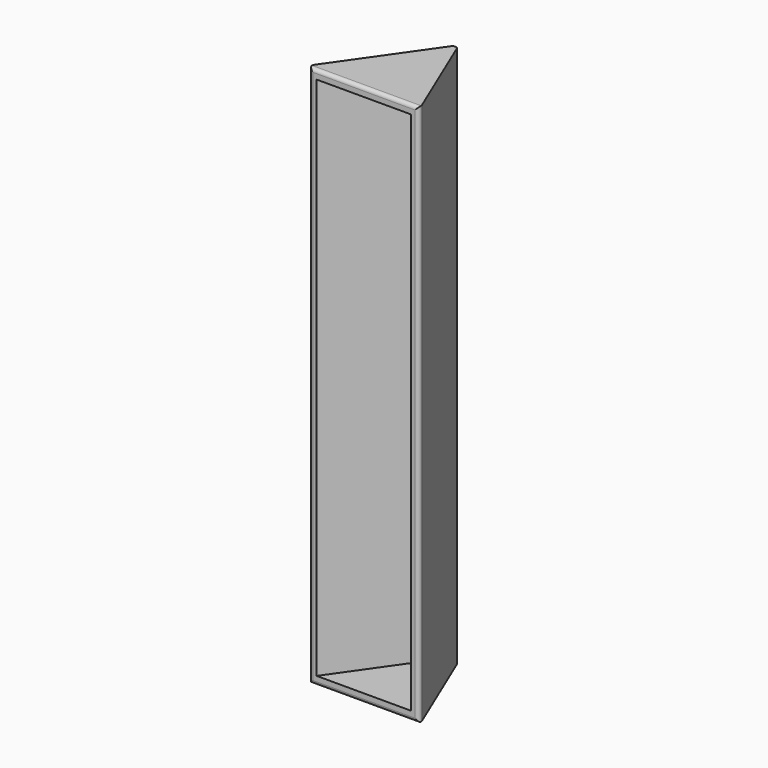
from build123d import *

# Parameters (mm, degrees)
F1_DEPTH      = 78.5
F2_T          = -2.5
F3_R          = 1
F4_TEXT_SIZE  = 12.5527115818
F5_DEPTH      = 1
F6_TEXT_SIZE  = 6.9016590714
F7_DEPTH      = 2
F8_TEXT_SIZE  = 8.8861462512
F9_DEPTH      = 1
F10_TEXT_SIZE = 8.2279131955
F11_DEPTH     = 0.5


# Not quite as in the source:
# - Text() gives the source's letters only with a copy of the font that has no kerning and outlines rounded to 1/6400 em; it was checked with that copy


with BuildPart() as f1:
    # F0 (on Top) → F1 (new body, symmetric)
    with BuildSketch(Plane.XY):
        Polygon((20.6212121212, 29.5087378695), (0, 0), (33, 0), align=None)
    extrude(amount=F1_DEPTH, both=True)

    # F2
    f2_openings = [f1.faces().sort_by_distance(p)[0] for p in [
        (16.5, 0, 0),
    ]]
    offset(amount=F2_T, openings=f2_openings)

    # F3
    f3_edges = [f1.edges().sort_by_distance(p)[0] for p in [
        (0, 0, 0),
        (20.621212, 29.508738, 0),
        (16.5, 0, -78.5),
        (33, 0, 0),
        (16.5, 0, 78.5),
    ]]
    fillet(f3_edges, radius=F3_R)

    # F4 (on face) → F5 (cut)
    with BuildSketch(Plane(origin=(0, 0, 0), x_dir=(-0.5728114478, -0.819687163, 0), z_dir=(-0.819687163, 0.5728114478, 0))):
        with Locations(Location((-11.6870761166, -13.866006701), (0, 0, 90))):
            Text('VIP 3D', F4_TEXT_SIZE, font='Open Sans', font_style=FontStyle.BOLD, text_align=(TextAlign.LEFT, TextAlign.BOTTOM))
    extrude(amount=-F5_DEPTH, mode=Mode.SUBTRACT)

    # F6 (on face) → F7 (join)
    with BuildSketch(Plane(origin=(0, 0, 0), x_dir=(-0.5728114478, -0.819687163, 0), z_dir=(-0.819687163, 0.5728114478, 0))):
        with Locations((-27.1170157939, -68.26813519)):
            Text('Vip 3D', F6_TEXT_SIZE, font='Open Sans', font_style=FontStyle.BOLD, text_align=(TextAlign.LEFT, TextAlign.BOTTOM))
    extrude(amount=F7_DEPTH)

    # F8 (on face) → F9 (join)
    with BuildSketch(Plane(origin=(0, 0, 0), x_dir=(-0.5728114478, -0.819687163, 0), z_dir=(-0.819687163, 0.5728114478, 0))):
        with Locations((-28.9187947777, -56.614848781)):
            Text('Vip 3d', F8_TEXT_SIZE, font='Open Sans', font_style=FontStyle.BOLD, text_align=(TextAlign.LEFT, TextAlign.BOTTOM))
    extrude(amount=F9_DEPTH)

    # F10 (on face) → F11 (join)
    with BuildSketch(Plane(origin=(0, 0, 0), x_dir=(-0.5728114478, -0.819687163, 0), z_dir=(-0.819687163, 0.5728114478, 0))):
        with Locations((-31.719027926, -46.1606789026)):
            Text('Vip 3d', F10_TEXT_SIZE, font='Open Sans', font_style=FontStyle.BOLD, text_align=(TextAlign.LEFT, TextAlign.BOTTOM))
    extrude(amount=F11_DEPTH)


solid = f1.part
